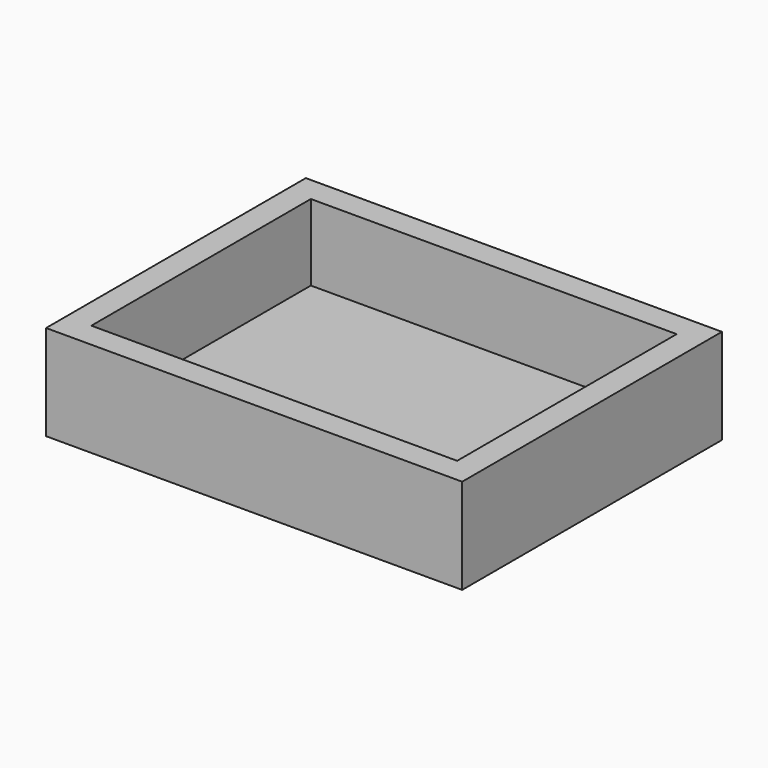
from build123d import *

# Parameters (mm, degrees)
F0_W     = 55.4736
F0_H     = 43.2816
F1_DEPTH = 12.7
F2_W     = 48.768
F2_H     = 36.576
F3_DEPTH = 10.16
F4_R     = 3.81
F5_DEPTH = 3.81


# Not quite as in the source:
# - a feature names something its author has since deleted; it is built from what else it names


with BuildPart() as f1:
    # F0 (on Top) → F1 (new body)
    with BuildSketch(Plane.XY):
        Rectangle(F0_W, F0_H)
    extrude(amount=F1_DEPTH)

    # F2 (on face) → F3 (cut)
    with BuildSketch(Plane.XY.offset(12.7)):
        Rectangle(F2_W, F2_H)
    extrude(amount=-F3_DEPTH, mode=Mode.SUBTRACT)

    # F4 (on face) → F5 (join)
    with BuildSketch(Plane(origin=(0, 0, 0), x_dir=(1, 0, 0), z_dir=(0, 0, -1))):
        with Locations((15.24, -10.16)):
            Circle(F4_R)
        with Locations((-15.24, -10.16)):
            Circle(F4_R)
        with Locations((15.24, 10.16)):
            Circle(F4_R)
        with Locations((-15.24, 10.16)):
            Circle(F4_R)
    extrude(amount=F5_DEPTH)


solid = f1.part
